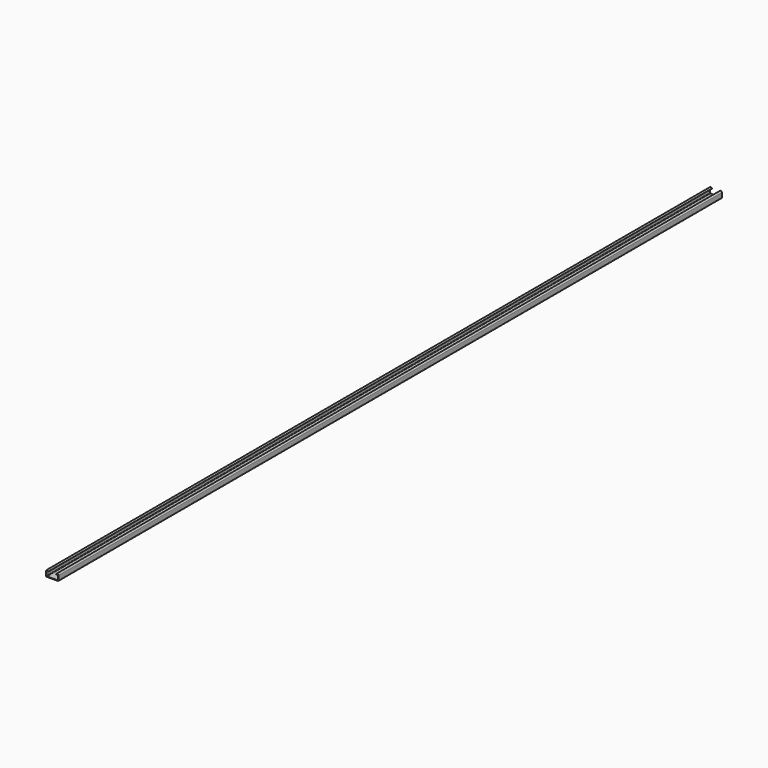
from build123d import *

# Parameters (mm, degrees)
F1_DEPTH    = 1381.125
F2_R        = 1.5875
F3_T1_DEPTH = 2767.5102424874
F3_T3_DEPTH = 2765.8360222341


# Not quite as in the source:
# - a fillet or chamfer that OpenCascade refuses, or shapes differently, is made with other operations: its cross-section is extruded or revolved along the edge and cut away or added


with BuildPart() as f1:
    # F0 (on Front) → F1 (new body, symmetric)
    with BuildSketch(Plane.XZ):
        with BuildLine():
            Line((0, 16.6624), (0, 0))
            Line((0, 0), (41.275, 0))
            Line((41.275, 0), (41.275, 16.6624))
            ThreePointArc((41.275, 16.6624), (37.3126, 20.6248), (33.3502, 16.6624))
            Line((33.3502, 16.6624), (34.9377, 16.6624))
            ThreePointArc((34.9377, 16.6624), (37.3126, 19.0373), (39.6875, 16.6624))
            Line((39.6875, 16.6624), (39.6875, 1.5875))
            Line((39.6875, 1.5875), (1.5875, 1.5875))
            Line((1.5875, 1.5875), (1.5875, 16.6624))
            ThreePointArc((1.5875, 16.6624), (3.9624, 19.0373), (6.3373, 16.6624))
            Line((6.3373, 16.6624), (7.9248, 16.6624))
            ThreePointArc((7.9248, 16.6624), (3.9624, 20.6248), (0, 16.6624))
        make_face()
    extrude(amount=F1_DEPTH, both=True)

    # F2
    f2_edges = [f1.edges().sort_by_distance(p)[0] for p in [
        (41.275, 0, 0),
        (0, 0, 0),
        (39.6875, 0, 1.5875),
        (1.5875, 0, 1.5875),
    ]]
    fillet(f2_edges, radius=F2_R)

    # F3: fillet of radius 0.8255 on 4 edges, made by hand

    # F3_s2 → F3_t1 (cut)
    with BuildSketch(Plane.XZ.offset(-1383.7551212437)):
        with BuildLine():
            ThreePointArc((7.7851364071, 17.7051368421), (7.6447738654, 16.9868405041), (6.9887329889, 16.6624))
            Line((6.9887329889, 16.6624), (7.9248, 16.6624))
            ThreePointArc((7.9248, 16.6624), (7.889728895, 17.1884242487), (7.7851364071, 17.7051368421))
        make_face()
        with BuildLine():
            ThreePointArc((33.4898635929, 17.7051368421), (33.6302261346, 16.9868405041), (34.2862670111, 16.6624))
            Line((34.2862670111, 16.6624), (33.3502, 16.6624))
            ThreePointArc((33.3502, 16.6624), (33.385271105, 17.1884242487), (33.4898635929, 17.7051368421))
        make_face()
    extrude(amount=F3_T1_DEPTH, mode=Mode.SUBTRACT)

    # F3_s4 → F3_t3 (cut)
    with BuildSketch(Plane.XZ.offset(-1382.918011117)):
        with BuildLine():
            ThreePointArc((6.2569378236, 17.2749734127), (6.551672789, 16.8332164322), (7.0545044468, 16.6624))
            Line((7.0545044468, 16.6624), (6.3373, 16.6624))
            ThreePointArc((6.3373, 16.6624), (6.317123751, 16.9713110978), (6.2569378236, 17.2749734127))
        make_face()
        with BuildLine():
            ThreePointArc((34.2204955532, 16.6624), (34.723327211, 16.8332164322), (35.0180621764, 17.2749734127))
            ThreePointArc((35.0180621764, 17.2749734127), (34.957876249, 16.9713110978), (34.9377, 16.6624))
            Line((34.9377, 16.6624), (34.2204955532, 16.6624))
        make_face()
    extrude(amount=F3_T3_DEPTH, mode=Mode.SUBTRACT)


solid = f1.part
